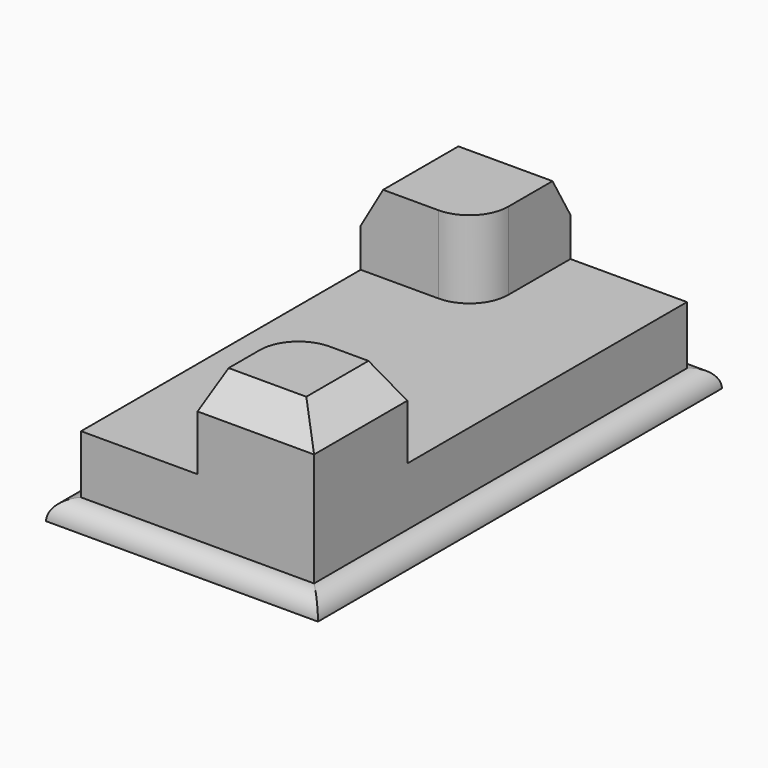
from build123d import *

# Parameters (mm, degrees)
F1_DEPTH = 50.8
F2_DEPTH = 25.4
F0_W     = 88.9
F0_H     = 165.1
F3_DEPTH = 6.35
F4_SIZE2 = 7.3323484187
F4_SIZE  = 12.7
F5_SIZE2 = 7.3323484187
F5_SIZE  = 12.7
F6_R     = 6.34999


# Not quite as in the source:
# - a fillet or chamfer is up to 0.001 mm smaller than in the source, because OpenCascade refuses the exact size


with BuildPart() as f1:
    # F0 (on Top) → F1 (new body)
    with BuildSketch(Plane.XY):
        with BuildLine():
            Line((2.826303332, 54.2691361523), (-35.273696668, 54.2691361523))
            Line((-35.273696668, 54.2691361523), (-35.273696668, 16.1691361523))
            Line((-35.273696668, 16.1691361523), (-9.873696668, 16.1691361523))
            ThreePointArc((-9.873696668, 16.1691361523), (-18.853952789, 37.8493922734), (2.826303332, 28.8691361523))
            Line((2.826303332, 28.8691361523), (2.826303332, 54.2691361523))
        make_face()
        with BuildLine():
            ThreePointArc((-9.873696668, 16.1691361523), (-0.8934405469, 19.8888800313), (2.826303332, 28.8691361523))
            ThreePointArc((2.826303332, 28.8691361523), (-18.853952789, 37.8493922734), (-9.873696668, 16.1691361523))
        make_face()
    extrude(amount=F1_DEPTH)

    # F5
    f5_edges = [f1.edges().sort_by_distance(p)[0] for p in [
        (-16.223697, 54.269136, 50.8),
        (-35.273697, 35.219136, 50.8),
    ]]
    chamfer(f5_edges, length=F5_SIZE, length2=F5_SIZE2)


with BuildPart() as f1b:
    # F0 (on Top) → F1, piece 2 (new body)
    with BuildSketch(Plane.XY):
        with BuildLine():
            ThreePointArc((28.226303332, -72.7308638477), (24.5065594531, -63.7506077266), (15.526303332, -60.0308638477))
            ThreePointArc((15.526303332, -60.0308638477), (6.546047211, -63.7506077266), (2.826303332, -72.7308638477))
            ThreePointArc((2.826303332, -72.7308638477), (15.526303332, -85.4308638477), (28.226303332, -72.7308638477))
        make_face()
        with BuildLine():
            Line((40.926303332, -98.1308638477), (40.926303332, -60.0308638477))
            Line((40.926303332, -60.0308638477), (15.526303332, -60.0308638477))
            ThreePointArc((15.526303332, -60.0308638477), (24.5065594531, -63.7506077266), (28.226303332, -72.7308638477))
            ThreePointArc((28.226303332, -72.7308638477), (15.526303332, -85.4308638477), (2.826303332, -72.7308638477))
            Line((2.826303332, -72.7308638477), (2.826303332, -98.1308638477))
            Line((2.826303332, -98.1308638477), (40.926303332, -98.1308638477))
        make_face()
    extrude(amount=F1_DEPTH)

    # F0 (on Top) → F2 (join)
    with BuildSketch(Plane.XY):
        with BuildLine():
            Line((40.926303332, 54.2691361523), (2.826303332, 54.2691361523))
            Line((2.826303332, 54.2691361523), (2.826303332, 28.8691361523))
            ThreePointArc((2.826303332, 28.8691361523), (-0.8934405469, 19.8888800313), (-9.873696668, 16.1691361523))
            Line((-9.873696668, 16.1691361523), (-35.273696668, 16.1691361523))
            Line((-35.273696668, 16.1691361523), (-35.273696668, -98.1308638477))
            Line((-35.273696668, -98.1308638477), (2.826303332, -98.1308638477))
            Line((2.826303332, -98.1308638477), (2.826303332, -72.7308638477))
            ThreePointArc((2.826303332, -72.7308638477), (6.546047211, -63.7506077266), (15.526303332, -60.0308638477))
            Line((15.526303332, -60.0308638477), (40.926303332, -60.0308638477))
            Line((40.926303332, -60.0308638477), (40.926303332, 54.2691361523))
        make_face()
    extrude(amount=F2_DEPTH)

    # F4
    f4_edges = [f1b.edges().sort_by_distance(p)[0] for p in [
        (21.876303, -98.130864, 50.8),
        (40.926303, -79.080864, 50.8),
    ]]
    f4_side = f1b.faces().sort_by_distance((22.272346, -79.476906, 50.8))[0]
    chamfer(f4_edges, length=F4_SIZE, length2=F4_SIZE2, reference=f4_side)


with BuildPart() as f3:
    # F0 (on Top) → F3 (new body)
    with BuildSketch(Plane.XY):
        with Locations((2.826303332, -21.9308638477)):
            Rectangle(F0_W, F0_H)
        Polygon((-35.273696668, 16.1691361523), (-35.273696668, 54.2691361523), (2.826303332, 54.2691361523), (40.926303332, 54.2691361523), (40.926303332, -60.0308638477), (40.926303332, -98.1308638477), (2.826303332, -98.1308638477), (-35.273696668, -98.1308638477), align=None, mode=Mode.SUBTRACT)
    extrude(amount=F3_DEPTH)

    # F6 (radius 6.35 in the source; OpenCascade refuses exactly that, so slightly less here)
    f6_edges = [f3.edges().sort_by_distance(p)[0] for p in [
        (47.276303, -21.930864, 6.35),
        (2.826303, 60.619136, 6.35),
        (-41.623697, -21.930864, 6.35),
        (2.826303, -104.480864, 6.35),
    ]]
    fillet(f6_edges, radius=F6_R)


solid = Compound([f1.part, f1b.part, f3.part])
